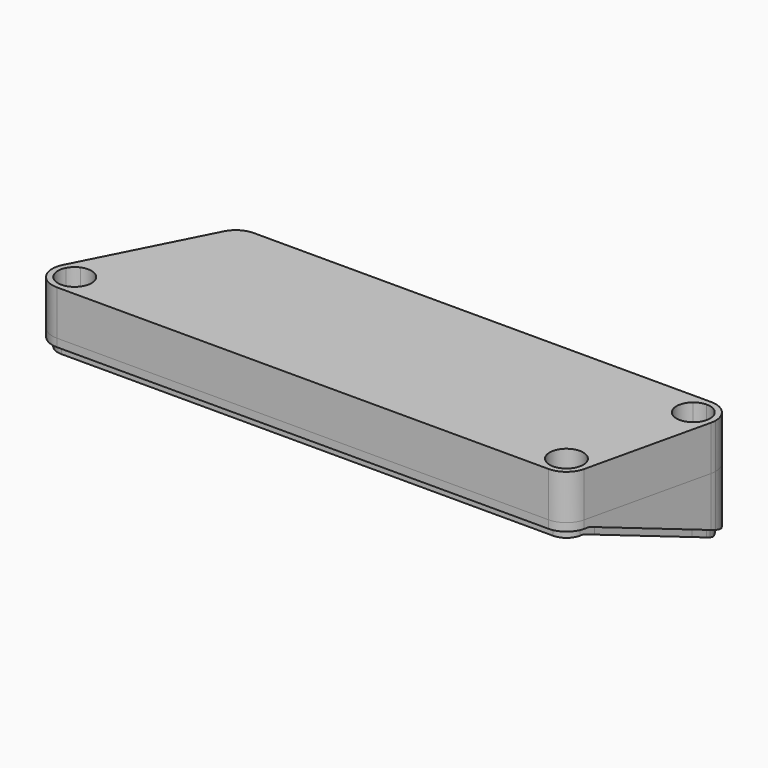
from build123d import *

# Parameters (mm, degrees)
F0_R           = 1.5
F1_DEPTH       = 8
F2_START       = 7
F2_DEPTH       = 1
F3_DEPTH       = 11
F4_DEPTH       = 11
F6_DEPTH       = 49.7516412236
F6_DEPTH_BACK  = 51.2503587764
F7_DEPTH       = 49.7516412236
F7_DEPTH_BACK  = 51.2503587764
F8_START       = 2
F8_DEPTH       = 6.001
F9_DEPTH       = 25
F9_DEPTH_BACK  = 5.5
F10_DEPTH      = 11.001
F10_DEPTH_BACK = 8.001


# Not quite as in the source:
# - a feature names something its author has since deleted; it is built from what else it names


with BuildPart() as f1:
    # F0 (on Top) → F1 (new body)
    with BuildSketch(Plane.XY):
        with BuildLine():
            Line((-38.1051070885, 12.8159626721), (-49.3146686248, -9.1840405611))
            ThreePointArc((-49.3146686248, -9.1840405611), (-48.4424439072, -8.0412505492), (-47.2225148362, -7.2806468212))
            Line((-47.2225148362, -7.2806468212), (-38.4152468672, 10.0045898197))
            ThreePointArc((-38.4152468672, 10.0045898197), (-38.5169619581, 11.4386037716), (-38.1051070885, 12.8159626721))
        make_face()
        with BuildLine():
            ThreePointArc((-47.2225148362, -7.2806468212), (-48.4424439072, -8.0412505492), (-49.3146686248, -9.1840405611))
            ThreePointArc((-49.3146686248, -9.1840405611), (-49.1612011474, -13.0899954561), (-45.7506412886, -15))
            ThreePointArc((-45.7506412886, -15), (-44.3364276916, -14.7416573983), (-43.1048899125, -14))
            Line((-43.1048899125, -14), (-45.7506412236, -14))
            ThreePointArc((-45.7506412236, -14), (-48.3085617166, -12.5674956941), (-48.4236607961, -9.6380285008))
            Line((-48.4236607961, -9.6380285008), (-47.2225148362, -7.2806468212))
        make_face()
        with BuildLine():
            ThreePointArc((-43.1048899125, -14), (-44.3364276916, -14.7416573983), (-45.7506412886, -15))
            Line((-45.7506412886, -15), (42.1702585717, -15))
            ThreePointArc((42.1702585717, -15), (40.7560450093, -14.7416573868), (39.5245072606, -14))
            Line((39.5245072606, -14), (-43.1048899125, -14))
        make_face()
        with BuildLine():
            ThreePointArc((-34.5410813347, 15), (-36.6310752715, 14.4105608548), (-38.1051070885, 12.8159626721))
            ThreePointArc((-38.1051070885, 12.8159626721), (-38.5169619581, 11.4386037716), (-38.4152468672, 10.0045898197))
            Line((-38.4152468672, 10.0045898197), (-37.2141009073, 12.3619714992))
            ThreePointArc((-37.2141009073, 12.3619714992), (-36.1085770289, 13.5579204931), (-34.5410813347, 14))
            Line((-34.5410813347, 14), (-31.8953300236, 14))
            ThreePointArc((-31.8953300236, 14), (-33.1268677723, 14.7416573868), (-34.5410813347, 15))
        make_face()
        with BuildLine():
            Line((-38.4152468672, 10.0045898197), (-47.2225148362, -7.2806468212))
            ThreePointArc((-47.2225148362, -7.2806468212), (-46.7754616454, -7.133510235), (-46.3142207299, -7.0399017512))
            Line((-46.3142207299, -7.0399017512), (-38.0761318397, 9.12825805))
            ThreePointArc((-38.0761318397, 9.12825805), (-38.2715115934, 9.5564314755), (-38.4152468672, 10.0045898197))
        make_face()
        with BuildLine():
            ThreePointArc((-46.3142207299, -7.0399017512), (-46.7754616454, -7.133510235), (-47.2225148362, -7.2806468212))
            Line((-47.2225148362, -7.2806468212), (-48.4236607961, -9.6380285008))
            ThreePointArc((-48.4236607961, -9.6380285008), (-47.7976986116, -8.8069299942), (-46.9255087711, -8.2396220828))
            Line((-46.9255087711, -8.2396220828), (-46.3142207299, -7.0399017512))
        make_face()
        with BuildLine():
            ThreePointArc((39.5245072606, -14), (40.7560450093, -14.7416573868), (42.1702585717, -15))
            ThreePointArc((42.1702585717, -15), (44.6603169083, -14.1304327943), (46.0677387101, -11.89980474))
            ThreePointArc((46.0677387101, -11.89980474), (46.144545964, -11.4528131215), (46.1702585717, -11))
            ThreePointArc((46.1702585717, -11), (46.047957565, -10.0184448475), (45.688533313, -9.0969122867))
            Line((45.688533313, -9.0969122867), (45.093368766, -11.674853163))
            ThreePointArc((45.093368766, -11.674853163), (44.0378024816, -13.3478244706), (42.1702585717, -14))
            Line((42.1702585717, -14), (39.5245072606, -14))
        make_face()
        with BuildLine():
            Line((-45.7506412236, -14), (-43.1048899125, -14))
            ThreePointArc((-43.1048899125, -14), (-42.7708323527, -13.6684713027), (-42.4780275892, -13.3))
            Line((-42.4780275892, -13.3), (-43.8245051952, -13.3))
            ThreePointArc((-43.8245051952, -13.3), (-44.725946147, -13.819574436), (-45.7506412236, -14))
        make_face()
        with BuildLine():
            ThreePointArc((-42.4780275892, -13.3), (-42.7708323527, -13.6684713027), (-43.1048899125, -14))
            Line((-43.1048899125, -14), (39.5245072606, -14))
            ThreePointArc((39.5245072606, -14), (39.1904497008, -13.6684713027), (38.8976449373, -13.3))
            Line((38.8976449373, -13.3), (-42.4780275892, -13.3))
        make_face()
        with BuildLine():
            Line((47.2493587764, 15), (-34.5410813347, 15))
            ThreePointArc((-34.5410813347, 15), (-33.1268677723, 14.7416573868), (-31.8953300236, 14))
            Line((-31.8953300236, 14), (44.6036074654, 14))
            ThreePointArc((44.6036074654, 14), (45.835145214, 14.7416573868), (47.2493587764, 15))
        make_face()
        with BuildLine():
            Line((-37.2141009073, 12.3619714992), (-38.4152468672, 10.0045898197))
            ThreePointArc((-38.4152468672, 10.0045898197), (-38.2715115934, 9.5564314755), (-38.0761318397, 9.12825805))
            Line((-38.0761318397, 9.12825805), (-37.4648437984, 10.3279783816))
            ThreePointArc((-37.4648437984, 10.3279783816), (-37.5185423825, 11.3670500087), (-37.2141009073, 12.3619714992))
        make_face()
        with BuildLine():
            ThreePointArc((-41.7506412236, -11), (-43.129030843, -7.9788811654), (-46.3142207299, -7.0399017512))
            Line((-46.3142207299, -7.0399017512), (-46.9255087711, -8.2396220828))
            ThreePointArc((-46.9255087711, -8.2396220828), (-44.0960419734, -8.4975409451), (-42.7506412236, -11))
            ThreePointArc((-42.7506412236, -11), (-43.0323321825, -12.2691713664), (-43.8245051952, -13.3))
            Line((-43.8245051952, -13.3), (-42.4780275892, -13.3))
            ThreePointArc((-42.4780275892, -13.3), (-41.9368206629, -12.2061395986), (-41.7506412236, -11))
        make_face()
        with BuildLine():
            ThreePointArc((-46.9255087711, -8.2396220828), (-47.7976986116, -8.8069299942), (-48.4236607961, -9.6380285008))
            ThreePointArc((-48.4236607961, -9.6380285008), (-48.3085617166, -12.5674956941), (-45.7506412236, -14))
            ThreePointArc((-45.7506412236, -14), (-44.725946147, -13.819574436), (-43.8245051952, -13.3))
            ThreePointArc((-43.8245051952, -13.3), (-43.0323321825, -12.2691713664), (-42.7506412236, -11))
            ThreePointArc((-42.7506412236, -11), (-44.0960419734, -8.4975409451), (-46.9255087711, -8.2396220828))
        make_face()
        with Locations((-45.7506412236, -11)):
            Circle(F0_R, mode=Mode.SUBTRACT)
        with BuildLine():
            ThreePointArc((38.8976449373, -13.3), (39.1904497008, -13.6684713027), (39.5245072606, -14))
            Line((39.5245072606, -14), (42.1702585717, -14))
            ThreePointArc((42.1702585717, -14), (41.1455634951, -13.819574436), (40.2441225432, -13.3))
            Line((40.2441225432, -13.3), (38.8976449373, -13.3))
        make_face()
        with BuildLine():
            ThreePointArc((46.1702585717, -11), (46.144545964, -11.4528131215), (46.0677387101, -11.89980474))
            Line((46.0677387101, -11.89980474), (51.1468383433, 10.1001927841))
            ThreePointArc((51.1468383433, 10.1001927841), (50.576988041, 8.7803415854), (49.5773044238, 7.7472059606))
            Line((49.5773044238, 7.7472059606), (45.688533313, -9.0969122867))
            ThreePointArc((45.688533313, -9.0969122867), (46.047957565, -10.0184448475), (46.1702585717, -11))
        make_face()
        with BuildLine():
            ThreePointArc((51.2493587764, 11), (50.0777859012, 13.8284271247), (47.2493587764, 15))
            ThreePointArc((47.2493587764, 15), (45.835145214, 14.7416573868), (44.6036074654, 14))
            Line((44.6036074654, 14), (47.2493587764, 14))
            ThreePointArc((47.2493587764, 14), (49.37067912, 13.1213203436), (50.2493587764, 11))
            ThreePointArc((50.2493587764, 11), (50.2300743435, 10.6603903587), (50.1724689708, 10.325146837))
            Line((50.1724689708, 10.325146837), (49.5773044238, 7.7472059606))
            ThreePointArc((49.5773044238, 7.7472059606), (50.576988041, 8.7803415854), (51.1468383433, 10.1001927841))
            ThreePointArc((51.1468383433, 10.1001927841), (51.2236460249, 10.5471856161), (51.2493587764, 11))
        make_face()
        with BuildLine():
            Line((44.6036074654, 14), (-31.8953300236, 14))
            ThreePointArc((-31.8953300236, 14), (-31.5612724638, 13.6684713027), (-31.2684677003, 13.3))
            Line((-31.2684677003, 13.3), (43.976745142, 13.3))
            ThreePointArc((43.976745142, 13.3), (44.2695499056, 13.6684713027), (44.6036074654, 14))
        make_face()
        with BuildLine():
            ThreePointArc((-31.2684677003, 13.3), (-31.5612724638, 13.6684713027), (-31.8953300236, 14))
            Line((-31.8953300236, 14), (-34.5410813347, 14))
            ThreePointArc((-34.5410813347, 14), (-33.5163862581, 13.819574436), (-32.6149453063, 13.3))
            Line((-32.6149453063, 13.3), (-31.2684677003, 13.3))
        make_face()
        with BuildLine():
            ThreePointArc((-34.5410813347, 14), (-36.1085770289, 13.5579204931), (-37.2141009073, 12.3619714992))
            ThreePointArc((-37.2141009073, 12.3619714992), (-37.5185423825, 11.3670500087), (-37.4648437984, 10.3279783816))
            Line((-37.4648437984, 10.3279783816), (-36.590396089, 12.0441786426))
            Line((-36.590396089, 12.0441786426), (-35.9505231474, 13.3))
            Line((-35.9505231474, 13.3), (-34.5410813347, 13.3))
            Line((-34.5410813347, 13.3), (-32.6149453063, 13.3))
            ThreePointArc((-32.6149453063, 13.3), (-33.5163862581, 13.819574436), (-34.5410813347, 14))
        make_face()
        with BuildLine():
            ThreePointArc((45.1474876082, -8.328650666), (39.6802000251, -7.8695673726), (38.8976449373, -13.3))
            Line((38.8976449373, -13.3), (40.2441225432, -13.3))
            ThreePointArc((40.2441225432, -13.3), (40.3027146617, -8.6521755294), (44.8445960511, -9.6406181382))
            Line((44.8445960511, -9.6406181382), (45.1474876082, -8.328650666))
        make_face()
        with BuildLine():
            ThreePointArc((40.2441225432, -13.3), (41.1455634951, -13.819574436), (42.1702585717, -14))
            ThreePointArc((42.1702585717, -14), (44.0378024816, -13.3478244706), (45.093368766, -11.674853163))
            ThreePointArc((45.093368766, -11.674853163), (45.1509741387, -11.3396096413), (45.1702585717, -11))
            ThreePointArc((45.1702585717, -11), (45.087707152, -10.3010766989), (44.8445960511, -9.6406181382))
            ThreePointArc((44.8445960511, -9.6406181382), (40.3027146617, -8.6521755294), (40.2441225432, -13.3))
        make_face()
        with Locations((42.1702585717, -11)):
            Circle(F0_R, mode=Mode.SUBTRACT)
        with BuildLine():
            Line((47.2493587764, 14), (44.6036074654, 14))
            ThreePointArc((44.6036074654, 14), (44.2695499056, 13.6684713027), (43.976745142, 13.3))
            Line((43.976745142, 13.3), (45.323222748, 13.3))
            ThreePointArc((45.323222748, 13.3), (46.2246636998, 13.819574436), (47.2493587764, 14))
        make_face()
        with BuildLine():
            Line((48.7542320379, 7.2938758161), (45.1474876082, -8.328650666))
            ThreePointArc((45.1474876082, -8.328650666), (45.4406482749, -8.6968388705), (45.688533313, -9.0969122867))
            Line((45.688533313, -9.0969122867), (49.5773044238, 7.7472059606))
            ThreePointArc((49.5773044238, 7.7472059606), (49.1791261852, 7.4962880044), (48.7542320379, 7.2938758161))
        make_face()
        with BuildLine():
            ThreePointArc((45.688533313, -9.0969122867), (45.4406482749, -8.6968388705), (45.1474876082, -8.328650666))
            Line((45.1474876082, -8.328650666), (44.8445960511, -9.6406181382))
            ThreePointArc((44.8445960511, -9.6406181382), (45.087707152, -10.3010766989), (45.1702585717, -11))
            ThreePointArc((45.1702585717, -11), (45.1509741387, -11.3396096413), (45.093368766, -11.674853163))
            Line((45.093368766, -11.674853163), (45.688533313, -9.0969122867))
        make_face()
        with BuildLine():
            ThreePointArc((48.7542320379, 7.2938758161), (49.1791261852, 7.4962880044), (49.5773044238, 7.7472059606))
            Line((49.5773044238, 7.7472059606), (50.1724689708, 10.325146837))
            ThreePointArc((50.1724689708, 10.325146837), (49.7661614644, 9.3673015497), (49.057123595, 8.6058432882))
            Line((49.057123595, 8.6058432882), (48.7542320379, 7.2938758161))
        make_face()
        with BuildLine():
            Line((45.323222748, 13.3), (43.976745142, 13.3))
            ThreePointArc((43.976745142, 13.3), (44.118926149, 8.5099414534), (48.7542320379, 7.2938758161))
            Line((48.7542320379, 7.2938758161), (49.057123595, 8.6058432882))
            ThreePointArc((49.057123595, 8.6058432882), (44.9015343059, 9.1324560901), (45.323222748, 13.3))
        make_face()
        with BuildLine():
            ThreePointArc((50.2493587764, 11), (49.37067912, 13.1213203436), (47.2493587764, 14))
            ThreePointArc((47.2493587764, 14), (46.2246636998, 13.819574436), (45.323222748, 13.3))
            ThreePointArc((45.323222748, 13.3), (44.9015343059, 9.1324560901), (49.057123595, 8.6058432882))
            ThreePointArc((49.057123595, 8.6058432882), (49.7661614644, 9.3673015497), (50.1724689708, 10.325146837))
            ThreePointArc((50.1724689708, 10.325146837), (50.2300743435, 10.6603903587), (50.2493587764, 11))
        make_face()
        with Locations((47.2493587764, 11)):
            Circle(F0_R, mode=Mode.SUBTRACT)
        with BuildLine():
            Line((-35.9505231474, 13.3), (-36.590396089, 12.0441786426))
            ThreePointArc((-36.590396089, 12.0441786426), (-35.7428277976, 12.9610725226), (-34.5410813347, 13.3))
            Line((-34.5410813347, 13.3), (-35.9505231474, 13.3))
        make_face()
        with Locations((47.2493587764, 11)):
            Circle(F0_R)
        with Locations((42.1702585717, -11)):
            Circle(F0_R)
    extrude(amount=F1_DEPTH)

    # F0 (on Top) → F2 (join)
    with BuildSketch(Plane.XY.offset(F2_START)):
        with BuildLine():
            Line((-38.0761318397, 9.12825805), (-46.3142207299, -7.0399017512))
            ThreePointArc((-46.3142207299, -7.0399017512), (-43.129030843, -7.9788811654), (-41.7506412236, -11))
            ThreePointArc((-41.7506412236, -11), (-41.9368206629, -12.2061395986), (-42.4780275892, -13.3))
            Line((-42.4780275892, -13.3), (38.8976449373, -13.3))
            ThreePointArc((38.8976449373, -13.3), (39.6802000251, -7.8695673726), (45.1474876082, -8.328650666))
            Line((45.1474876082, -8.328650666), (48.7542320379, 7.2938758161))
            ThreePointArc((48.7542320379, 7.2938758161), (44.118926149, 8.5099414534), (43.976745142, 13.3))
            Line((43.976745142, 13.3), (-31.2684677003, 13.3))
            ThreePointArc((-31.2684677003, 13.3), (-30.7272607741, 12.2061395986), (-30.5410813347, 11))
            ThreePointArc((-30.5410813347, 11), (-33.5767686312, 7.1179772013), (-38.0761318397, 9.12825805))
        make_face()
        with BuildLine():
            Line((-36.590396089, 12.0441786426), (-37.4648437984, 10.3279783816))
            ThreePointArc((-37.4648437984, 10.3279783816), (-34.2029152448, 8.0191203151), (-31.5410813347, 11))
            ThreePointArc((-31.5410813347, 11), (-31.8227722937, 12.2691713664), (-32.6149453063, 13.3))
            Line((-32.6149453063, 13.3), (-34.5410813347, 13.3))
            ThreePointArc((-34.5410813347, 13.3), (-32.914735738, 12.6263455967), (-32.2410813347, 11))
            ThreePointArc((-32.2410813347, 11), (-35.0780059407, 8.7635492477), (-36.590396089, 12.0441786426))
        make_face()
        with BuildLine():
            ThreePointArc((-34.5410813347, 13.3), (-35.7428277976, 12.9610725226), (-36.590396089, 12.0441786426))
            ThreePointArc((-36.590396089, 12.0441786426), (-35.0780059407, 8.7635492477), (-32.2410813347, 11))
            ThreePointArc((-32.2410813347, 11), (-32.914735738, 12.6263455967), (-34.5410813347, 13.3))
        make_face()
        with Locations((-34.5410813347, 11)):
            Circle(F0_R, mode=Mode.SUBTRACT)
        with Locations((-34.5410813347, 11)):
            Circle(F0_R)
        with BuildLine():
            Line((-37.4648437984, 10.3279783816), (-38.0761318397, 9.12825805))
            ThreePointArc((-38.0761318397, 9.12825805), (-33.5767686312, 7.1179772013), (-30.5410813347, 11))
            ThreePointArc((-30.5410813347, 11), (-30.7272607741, 12.2061395986), (-31.2684677003, 13.3))
            Line((-31.2684677003, 13.3), (-32.6149453063, 13.3))
            ThreePointArc((-32.6149453063, 13.3), (-31.8227722937, 12.2691713664), (-31.5410813347, 11))
            ThreePointArc((-31.5410813347, 11), (-34.2029152448, 8.0191203151), (-37.4648437984, 10.3279783816))
        make_face()
    extrude(amount=F2_DEPTH)

    # F0 (on Top) → F3 (join)
    with BuildSketch(Plane.XY):
        with BuildLine():
            ThreePointArc((-42.4780275892, -13.3), (-42.7708323527, -13.6684713027), (-43.1048899125, -14))
            Line((-43.1048899125, -14), (39.5245072606, -14))
            ThreePointArc((39.5245072606, -14), (39.1904497008, -13.6684713027), (38.8976449373, -13.3))
            Line((38.8976449373, -13.3), (-42.4780275892, -13.3))
        make_face()
        with BuildLine():
            Line((44.6036074654, 14), (-31.8953300236, 14))
            ThreePointArc((-31.8953300236, 14), (-31.5612724638, 13.6684713027), (-31.2684677003, 13.3))
            Line((-31.2684677003, 13.3), (43.976745142, 13.3))
            ThreePointArc((43.976745142, 13.3), (44.2695499056, 13.6684713027), (44.6036074654, 14))
        make_face()
        with BuildLine():
            ThreePointArc((-46.9255087711, -8.2396220828), (-47.7976986116, -8.8069299942), (-48.4236607961, -9.6380285008))
            ThreePointArc((-48.4236607961, -9.6380285008), (-48.3085617166, -12.5674956941), (-45.7506412236, -14))
            ThreePointArc((-45.7506412236, -14), (-44.725946147, -13.819574436), (-43.8245051952, -13.3))
            ThreePointArc((-43.8245051952, -13.3), (-43.0323321825, -12.2691713664), (-42.7506412236, -11))
            ThreePointArc((-42.7506412236, -11), (-44.0960419734, -8.4975409451), (-46.9255087711, -8.2396220828))
        make_face()
        with Locations((-45.7506412236, -11)):
            Circle(F0_R, mode=Mode.SUBTRACT)
        with BuildLine():
            ThreePointArc((50.2493587764, 11), (49.37067912, 13.1213203436), (47.2493587764, 14))
            ThreePointArc((47.2493587764, 14), (46.2246636998, 13.819574436), (45.323222748, 13.3))
            ThreePointArc((45.323222748, 13.3), (44.9015343059, 9.1324560901), (49.057123595, 8.6058432882))
            ThreePointArc((49.057123595, 8.6058432882), (49.7661614644, 9.3673015497), (50.1724689708, 10.325146837))
            ThreePointArc((50.1724689708, 10.325146837), (50.2300743435, 10.6603903587), (50.2493587764, 11))
        make_face()
        with Locations((47.2493587764, 11)):
            Circle(F0_R, mode=Mode.SUBTRACT)
        with BuildLine():
            ThreePointArc((40.2441225432, -13.3), (41.1455634951, -13.819574436), (42.1702585717, -14))
            ThreePointArc((42.1702585717, -14), (44.0378024816, -13.3478244706), (45.093368766, -11.674853163))
            ThreePointArc((45.093368766, -11.674853163), (45.1509741387, -11.3396096413), (45.1702585717, -11))
            ThreePointArc((45.1702585717, -11), (45.087707152, -10.3010766989), (44.8445960511, -9.6406181382))
            ThreePointArc((44.8445960511, -9.6406181382), (40.3027146617, -8.6521755294), (40.2441225432, -13.3))
        make_face()
        with Locations((42.1702585717, -11)):
            Circle(F0_R, mode=Mode.SUBTRACT)
        with BuildLine():
            Line((-38.4152468672, 10.0045898197), (-47.2225148362, -7.2806468212))
            ThreePointArc((-47.2225148362, -7.2806468212), (-46.7754616454, -7.133510235), (-46.3142207299, -7.0399017512))
            Line((-46.3142207299, -7.0399017512), (-38.0761318397, 9.12825805))
            ThreePointArc((-38.0761318397, 9.12825805), (-38.2715115934, 9.5564314755), (-38.4152468672, 10.0045898197))
        make_face()
        with BuildLine():
            Line((48.7542320379, 7.2938758161), (45.1474876082, -8.328650666))
            ThreePointArc((45.1474876082, -8.328650666), (45.4406482749, -8.6968388705), (45.688533313, -9.0969122867))
            Line((45.688533313, -9.0969122867), (49.5773044238, 7.7472059606))
            ThreePointArc((49.5773044238, 7.7472059606), (49.1791261852, 7.4962880044), (48.7542320379, 7.2938758161))
        make_face()
        with BuildLine():
            ThreePointArc((45.1474876082, -8.328650666), (39.6802000251, -7.8695673726), (38.8976449373, -13.3))
            Line((38.8976449373, -13.3), (40.2441225432, -13.3))
            ThreePointArc((40.2441225432, -13.3), (40.3027146617, -8.6521755294), (44.8445960511, -9.6406181382))
            Line((44.8445960511, -9.6406181382), (45.1474876082, -8.328650666))
        make_face()
        with BuildLine():
            Line((45.323222748, 13.3), (43.976745142, 13.3))
            ThreePointArc((43.976745142, 13.3), (44.118926149, 8.5099414534), (48.7542320379, 7.2938758161))
            Line((48.7542320379, 7.2938758161), (49.057123595, 8.6058432882))
            ThreePointArc((49.057123595, 8.6058432882), (44.9015343059, 9.1324560901), (45.323222748, 13.3))
        make_face()
        with BuildLine():
            ThreePointArc((-41.7506412236, -11), (-43.129030843, -7.9788811654), (-46.3142207299, -7.0399017512))
            Line((-46.3142207299, -7.0399017512), (-46.9255087711, -8.2396220828))
            ThreePointArc((-46.9255087711, -8.2396220828), (-44.0960419734, -8.4975409451), (-42.7506412236, -11))
            ThreePointArc((-42.7506412236, -11), (-43.0323321825, -12.2691713664), (-43.8245051952, -13.3))
            Line((-43.8245051952, -13.3), (-42.4780275892, -13.3))
            ThreePointArc((-42.4780275892, -13.3), (-41.9368206629, -12.2061395986), (-41.7506412236, -11))
        make_face()
        with Locations((47.2493587764, 11)):
            Circle(F0_R)
        with Locations((42.1702585717, -11)):
            Circle(F0_R)
        with BuildLine():
            ThreePointArc((-34.5410813347, 14), (-36.1085770289, 13.5579204931), (-37.2141009073, 12.3619714992))
            ThreePointArc((-37.2141009073, 12.3619714992), (-37.5185423825, 11.3670500087), (-37.4648437984, 10.3279783816))
            Line((-37.4648437984, 10.3279783816), (-36.590396089, 12.0441786426))
            Line((-36.590396089, 12.0441786426), (-35.9505231474, 13.3))
            Line((-35.9505231474, 13.3), (-34.5410813347, 13.3))
            Line((-34.5410813347, 13.3), (-32.6149453063, 13.3))
            ThreePointArc((-32.6149453063, 13.3), (-33.5163862581, 13.819574436), (-34.5410813347, 14))
        make_face()
        with BuildLine():
            ThreePointArc((45.688533313, -9.0969122867), (45.4406482749, -8.6968388705), (45.1474876082, -8.328650666))
            Line((45.1474876082, -8.328650666), (44.8445960511, -9.6406181382))
            ThreePointArc((44.8445960511, -9.6406181382), (45.087707152, -10.3010766989), (45.1702585717, -11))
            ThreePointArc((45.1702585717, -11), (45.1509741387, -11.3396096413), (45.093368766, -11.674853163))
            Line((45.093368766, -11.674853163), (45.688533313, -9.0969122867))
        make_face()
        with BuildLine():
            ThreePointArc((38.8976449373, -13.3), (39.1904497008, -13.6684713027), (39.5245072606, -14))
            Line((39.5245072606, -14), (42.1702585717, -14))
            ThreePointArc((42.1702585717, -14), (41.1455634951, -13.819574436), (40.2441225432, -13.3))
            Line((40.2441225432, -13.3), (38.8976449373, -13.3))
        make_face()
        with BuildLine():
            Line((-45.7506412236, -14), (-43.1048899125, -14))
            ThreePointArc((-43.1048899125, -14), (-42.7708323527, -13.6684713027), (-42.4780275892, -13.3))
            Line((-42.4780275892, -13.3), (-43.8245051952, -13.3))
            ThreePointArc((-43.8245051952, -13.3), (-44.725946147, -13.819574436), (-45.7506412236, -14))
        make_face()
        with BuildLine():
            Line((-37.2141009073, 12.3619714992), (-38.4152468672, 10.0045898197))
            ThreePointArc((-38.4152468672, 10.0045898197), (-38.2715115934, 9.5564314755), (-38.0761318397, 9.12825805))
            Line((-38.0761318397, 9.12825805), (-37.4648437984, 10.3279783816))
            ThreePointArc((-37.4648437984, 10.3279783816), (-37.5185423825, 11.3670500087), (-37.2141009073, 12.3619714992))
        make_face()
        with BuildLine():
            ThreePointArc((48.7542320379, 7.2938758161), (49.1791261852, 7.4962880044), (49.5773044238, 7.7472059606))
            Line((49.5773044238, 7.7472059606), (50.1724689708, 10.325146837))
            ThreePointArc((50.1724689708, 10.325146837), (49.7661614644, 9.3673015497), (49.057123595, 8.6058432882))
            Line((49.057123595, 8.6058432882), (48.7542320379, 7.2938758161))
        make_face()
        with BuildLine():
            ThreePointArc((-46.3142207299, -7.0399017512), (-46.7754616454, -7.133510235), (-47.2225148362, -7.2806468212))
            Line((-47.2225148362, -7.2806468212), (-48.4236607961, -9.6380285008))
            ThreePointArc((-48.4236607961, -9.6380285008), (-47.7976986116, -8.8069299942), (-46.9255087711, -8.2396220828))
            Line((-46.9255087711, -8.2396220828), (-46.3142207299, -7.0399017512))
        make_face()
        with BuildLine():
            ThreePointArc((-31.2684677003, 13.3), (-31.5612724638, 13.6684713027), (-31.8953300236, 14))
            Line((-31.8953300236, 14), (-34.5410813347, 14))
            ThreePointArc((-34.5410813347, 14), (-33.5163862581, 13.819574436), (-32.6149453063, 13.3))
            Line((-32.6149453063, 13.3), (-31.2684677003, 13.3))
        make_face()
        with BuildLine():
            Line((47.2493587764, 14), (44.6036074654, 14))
            ThreePointArc((44.6036074654, 14), (44.2695499056, 13.6684713027), (43.976745142, 13.3))
            Line((43.976745142, 13.3), (45.323222748, 13.3))
            ThreePointArc((45.323222748, 13.3), (46.2246636998, 13.819574436), (47.2493587764, 14))
        make_face()
        with BuildLine():
            Line((-35.9505231474, 13.3), (-36.590396089, 12.0441786426))
            ThreePointArc((-36.590396089, 12.0441786426), (-35.7428277976, 12.9610725226), (-34.5410813347, 13.3))
            Line((-34.5410813347, 13.3), (-35.9505231474, 13.3))
        make_face()
    extrude(amount=-F3_DEPTH)


with BuildPart() as f4:
    # F0 (on Top) → F4 (new body)
    with BuildSketch(Plane.XY):
        with BuildLine():
            Line((-38.1051070885, 12.8159626721), (-49.3146686248, -9.1840405611))
            ThreePointArc((-49.3146686248, -9.1840405611), (-48.4424439072, -8.0412505492), (-47.2225148362, -7.2806468212))
            Line((-47.2225148362, -7.2806468212), (-38.4152468672, 10.0045898197))
            ThreePointArc((-38.4152468672, 10.0045898197), (-38.5169619581, 11.4386037716), (-38.1051070885, 12.8159626721))
        make_face()
        with BuildLine():
            Line((47.2493587764, 15), (-34.5410813347, 15))
            ThreePointArc((-34.5410813347, 15), (-33.1268677723, 14.7416573868), (-31.8953300236, 14))
            Line((-31.8953300236, 14), (44.6036074654, 14))
            ThreePointArc((44.6036074654, 14), (45.835145214, 14.7416573868), (47.2493587764, 15))
        make_face()
        with BuildLine():
            ThreePointArc((46.1702585717, -11), (46.144545964, -11.4528131215), (46.0677387101, -11.89980474))
            Line((46.0677387101, -11.89980474), (51.1468383433, 10.1001927841))
            ThreePointArc((51.1468383433, 10.1001927841), (50.576988041, 8.7803415854), (49.5773044238, 7.7472059606))
            Line((49.5773044238, 7.7472059606), (45.688533313, -9.0969122867))
            ThreePointArc((45.688533313, -9.0969122867), (46.047957565, -10.0184448475), (46.1702585717, -11))
        make_face()
        with BuildLine():
            ThreePointArc((39.5245072606, -14), (40.7560450093, -14.7416573868), (42.1702585717, -15))
            ThreePointArc((42.1702585717, -15), (44.6603169083, -14.1304327943), (46.0677387101, -11.89980474))
            ThreePointArc((46.0677387101, -11.89980474), (46.144545964, -11.4528131215), (46.1702585717, -11))
            ThreePointArc((46.1702585717, -11), (46.047957565, -10.0184448475), (45.688533313, -9.0969122867))
            Line((45.688533313, -9.0969122867), (45.093368766, -11.674853163))
            ThreePointArc((45.093368766, -11.674853163), (44.0378024816, -13.3478244706), (42.1702585717, -14))
            Line((42.1702585717, -14), (39.5245072606, -14))
        make_face()
        with BuildLine():
            ThreePointArc((-47.2225148362, -7.2806468212), (-48.4424439072, -8.0412505492), (-49.3146686248, -9.1840405611))
            ThreePointArc((-49.3146686248, -9.1840405611), (-49.1612011474, -13.0899954561), (-45.7506412886, -15))
            ThreePointArc((-45.7506412886, -15), (-44.3364276916, -14.7416573983), (-43.1048899125, -14))
            Line((-43.1048899125, -14), (-45.7506412236, -14))
            ThreePointArc((-45.7506412236, -14), (-48.3085617166, -12.5674956941), (-48.4236607961, -9.6380285008))
            Line((-48.4236607961, -9.6380285008), (-47.2225148362, -7.2806468212))
        make_face()
        with BuildLine():
            ThreePointArc((-43.1048899125, -14), (-44.3364276916, -14.7416573983), (-45.7506412886, -15))
            Line((-45.7506412886, -15), (42.1702585717, -15))
            ThreePointArc((42.1702585717, -15), (40.7560450093, -14.7416573868), (39.5245072606, -14))
            Line((39.5245072606, -14), (-43.1048899125, -14))
        make_face()
        with BuildLine():
            ThreePointArc((-34.5410813347, 15), (-36.6310752715, 14.4105608548), (-38.1051070885, 12.8159626721))
            ThreePointArc((-38.1051070885, 12.8159626721), (-38.5169619581, 11.4386037716), (-38.4152468672, 10.0045898197))
            Line((-38.4152468672, 10.0045898197), (-37.2141009073, 12.3619714992))
            ThreePointArc((-37.2141009073, 12.3619714992), (-36.1085770289, 13.5579204931), (-34.5410813347, 14))
            Line((-34.5410813347, 14), (-31.8953300236, 14))
            ThreePointArc((-31.8953300236, 14), (-33.1268677723, 14.7416573868), (-34.5410813347, 15))
        make_face()
        with BuildLine():
            ThreePointArc((51.2493587764, 11), (50.0777859012, 13.8284271247), (47.2493587764, 15))
            ThreePointArc((47.2493587764, 15), (45.835145214, 14.7416573868), (44.6036074654, 14))
            Line((44.6036074654, 14), (47.2493587764, 14))
            ThreePointArc((47.2493587764, 14), (49.37067912, 13.1213203436), (50.2493587764, 11))
            ThreePointArc((50.2493587764, 11), (50.2300743435, 10.6603903587), (50.1724689708, 10.325146837))
            Line((50.1724689708, 10.325146837), (49.5773044238, 7.7472059606))
            ThreePointArc((49.5773044238, 7.7472059606), (50.576988041, 8.7803415854), (51.1468383433, 10.1001927841))
            ThreePointArc((51.1468383433, 10.1001927841), (51.2236460249, 10.5471856161), (51.2493587764, 11))
        make_face()
    extrude(amount=-F4_DEPTH)


with BuildPart() as f6_tool:
    # F5 (on Right) → F6 (new body, two sides)
    with BuildSketch(Plane.YZ) as f6_sk:
        Polygon((-11, -2.9164742901), (-15, -2.9164742901), (-15, -21.2085042149), (15, -21.2085042149), (15, -12.1235571759), (12.815961999, -11.3501487566), align=None)
        Polygon((15, -11.3501487566), (12.815961999, -11.3501487566), (15, -12.1235571759), align=None)
    extrude(amount=-F6_DEPTH)
    extrude(f6_sk.sketch, amount=F6_DEPTH_BACK)


with BuildPart() as f1_1:
    add(f1.part)

    # F6: cut by f6_tool
    add(f6_tool.part, mode=Mode.SUBTRACT)

    # F0 (on Top) → F8 (cut)
    with BuildSketch(Plane.XY.offset(F8_START)):
        with BuildLine():
            ThreePointArc((40.2441225432, -13.3), (41.1455634951, -13.819574436), (42.1702585717, -14))
            ThreePointArc((42.1702585717, -14), (44.0378024816, -13.3478244706), (45.093368766, -11.674853163))
            ThreePointArc((45.093368766, -11.674853163), (45.1509741387, -11.3396096413), (45.1702585717, -11))
            ThreePointArc((45.1702585717, -11), (45.087707152, -10.3010766989), (44.8445960511, -9.6406181382))
            ThreePointArc((44.8445960511, -9.6406181382), (40.3027146617, -8.6521755294), (40.2441225432, -13.3))
        make_face()
        with Locations((42.1702585717, -11)):
            Circle(F0_R, mode=Mode.SUBTRACT)
        with BuildLine():
            ThreePointArc((-46.9255087711, -8.2396220828), (-47.7976986116, -8.8069299942), (-48.4236607961, -9.6380285008))
            ThreePointArc((-48.4236607961, -9.6380285008), (-48.3085617166, -12.5674956941), (-45.7506412236, -14))
            ThreePointArc((-45.7506412236, -14), (-44.725946147, -13.819574436), (-43.8245051952, -13.3))
            ThreePointArc((-43.8245051952, -13.3), (-43.0323321825, -12.2691713664), (-42.7506412236, -11))
            ThreePointArc((-42.7506412236, -11), (-44.0960419734, -8.4975409451), (-46.9255087711, -8.2396220828))
        make_face()
        with Locations((-45.7506412236, -11)):
            Circle(F0_R, mode=Mode.SUBTRACT)
    extrude(amount=F8_DEPTH, mode=Mode.SUBTRACT)

    # F0 (on Top) → F9 (cut, two sides)
    with BuildSketch(Plane.XY) as f9_sk:
        with BuildLine():
            ThreePointArc((50.2493587764, 11), (49.37067912, 13.1213203436), (47.2493587764, 14))
            ThreePointArc((47.2493587764, 14), (46.2246636998, 13.819574436), (45.323222748, 13.3))
            ThreePointArc((45.323222748, 13.3), (44.9015343059, 9.1324560901), (49.057123595, 8.6058432882))
            ThreePointArc((49.057123595, 8.6058432882), (49.7661614644, 9.3673015497), (50.1724689708, 10.325146837))
            ThreePointArc((50.1724689708, 10.325146837), (50.2300743435, 10.6603903587), (50.2493587764, 11))
        make_face()
        with Locations((47.2493587764, 11)):
            Circle(F0_R, mode=Mode.SUBTRACT)
    extrude(amount=F9_DEPTH, mode=Mode.SUBTRACT)
    extrude(f9_sk.sketch, amount=-F9_DEPTH_BACK, mode=Mode.SUBTRACT)

    # F0 (on Top) → F10 (cut, two sides)
    with BuildSketch(Plane.XY) as f10_sk:
        with BuildLine():
            Line((-36.9922844873, 15), (-38.1051070885, 12.8159626721))
            ThreePointArc((-38.1051070885, 12.8159626721), (-36.6310752715, 14.4105608548), (-34.5410813347, 15))
            Line((-34.5410813347, 15), (-36.9922844873, 15))
        make_face()
        with BuildLine():
            Line((-49.3146686248, -9.1840405611), (-52.2780479721, -15))
            Line((-52.2780479721, -15), (-45.7506412886, -15))
            ThreePointArc((-45.7506412886, -15), (-49.1612011474, -13.0899954561), (-49.3146686248, -9.1840405611))
        make_face()
        with Locations((42.1702585717, -11)):
            Circle(F0_R)
        with BuildLine():
            ThreePointArc((46.0677387101, -11.89980474), (44.6603169083, -14.1304327943), (42.1702585717, -15))
            Line((42.1702585717, -15), (45.3520022383, -15))
            Line((45.3520022383, -15), (46.0677387101, -11.89980474))
        make_face()
        with Locations((47.2493587764, 11)):
            Circle(F0_R)
        with BuildLine():
            Line((52.2780479721, 15), (47.2493587764, 15))
            ThreePointArc((47.2493587764, 15), (50.0777859012, 13.8284271247), (51.2493587764, 11))
            ThreePointArc((51.2493587764, 11), (51.2236460249, 10.5471856161), (51.1468383433, 10.1001927841))
            Line((51.1468383433, 10.1001927841), (52.2780479721, 15))
        make_face()
    extrude(amount=-F10_DEPTH, mode=Mode.SUBTRACT)
    extrude(f10_sk.sketch, amount=F10_DEPTH_BACK, mode=Mode.SUBTRACT)


with BuildPart() as f4_1:
    add(f4.part)

    # F6: cut by f6_tool
    add(f6_tool.part, mode=Mode.SUBTRACT)

    # F5 (on Right) → F7 (cut, two sides)
    with BuildSketch(Plane.YZ) as f7_sk:
        Polygon((-11, -1.4164742901), (-15, -1.4164742901), (-15, -1.5), (-11, -2.9164742901), (12.815961999, -11.3501487566), (15, -11.3501487566), (15, -10.6235571759), (12.815961999, -9.8501487566), align=None)
        Polygon((-11, -2.9164742901), (-15, -1.5), (-15, -2.9164742901), align=None)
        Polygon((15, -9.8501487566), (12.815961999, -9.8501487566), (15, -10.6235571759), align=None)
    extrude(amount=-F7_DEPTH, mode=Mode.SUBTRACT)
    extrude(f7_sk.sketch, amount=F7_DEPTH_BACK, mode=Mode.SUBTRACT)


solid = Compound([f1_1.part, f4_1.part])
